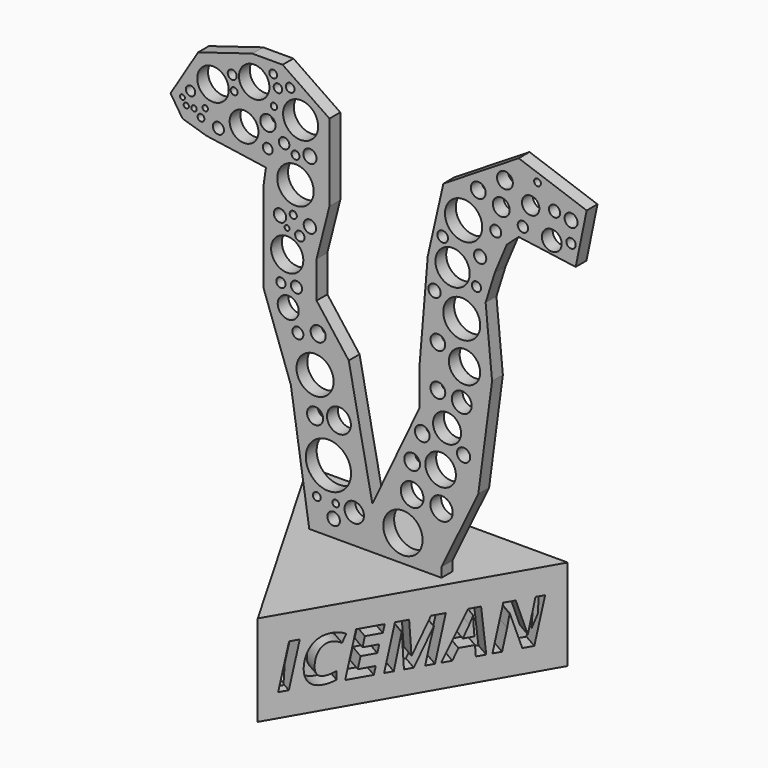
from build123d import *

# Parameters (mm, degrees)
F1_DEPTH     = 27
F2_TEXT_SIZE = 18.3817495487
F3_DEPTH     = 5
F4_TEXT_SIZE = 17.8425786241
F5_DEPTH     = 5
F6_TEXT_SIZE = 19.2699850433
F7_DEPTH     = 5
F9_DEPTH     = 127
F10_R        = 4.2621255768
F10_R_2      = 5.4056711116
F10_R_3      = 4.5113334329
F10_R_4      = 4.6639700848
F10_R_5      = 1.3923551174
F10_R_6      = 0.7328480671
F10_R_7      = 0.767759656
F10_R_8      = 0.8011609316
F10_R_9      = 1
F10_R_10     = 0.8092948289
F10_R_11     = 1.6459744272
F10_R_12     = 2.2704727082
F10_R_13     = 1.0363962707
F10_R_14     = 1.3396073613
F10_R_15     = 5.1942897194
F10_R_16     = 0.9437807842
F10_R_17     = 1.55798255
F10_R_18     = 1.4548048846
F10_R_19     = 1.1783421347
F10_R_20     = 1.9564498282
F10_R_21     = 1.0551848536
F10_R_22     = 1.8332824111
F10_R_23     = 0.7328445764
F10_R_24     = 1.392354505
F10_R_25     = 1.8332749605
F10_R_26     = 4.7727933339
F10_R_27     = 1.3781634382
F10_R_28     = 1.6454183226
F10_R_29     = 3.1159786158
F10_R_30     = 1.6266516452
F10_R_31     = 2.2244104358
F10_R_32     = 5.4998397827
F10_R_33     = 1.9248165419
F10_R_34     = 2.582420861
F10_R_35     = 1.5337907074
F10_R_36     = 2.5096557058
F10_R_37     = 2.1946331857
F10_R_38     = 5.5118577323
F10_R_39     = 5.0853234815
F10_R_40     = 1.5763342381
F10_R_41     = 1.822880463
F10_R_42     = 1.3610571623
F10_R_43     = 1.8260498017
F10_R_44     = 5.4713745158
F10_R_45     = 4.6355846875
F10_R_46     = 2.1776929498
F10_R_47     = 2.1946403477
F10_R_48     = 2.9317995196
F10_R_49     = 4.1461972463
F10_R_50     = 4.5304970367
F10_R_51     = 1.9629433151
F10_R_52     = 3.3115899201
F10_R_53     = 3.3670677037
F10_R_54     = 2.3408899759
F10_R_55     = 5.8192073402
F10_R_56     = 1.8585663298
F10_R_57     = 2.882521964
F10_R_58     = 0.9814695986
F10_R_59     = 1.1548921466
F10_R_60     = 6.7011643118
F10_R_61     = 2.3863964285
F10_R_62     = 3.5387465616
F10_R_63     = 2.3416440081
F10_R_64     = 1.6558003189
F10_R_65     = 2.9317919101
F10_R_66     = 1.3880112598
F10_R_67     = 1.633271575
F10_R_68     = 1.1445034295
F10_R_69     = 1.2597935008
F10_R_70     = 1.2796093116
F11_DEPTH    = 24.2289854638


# Not quite as in the source:
# - Text() gives the source's letters only with a copy of the font that has no kerning and outlines rounded to 1/6400 em; it was checked with that copy


with BuildPart() as f1:
    # F0 (on Top) → F1 (new body)
    with BuildSketch(Plane.XY):
        Polygon((38.5, 22.2279853638), (-38.5, 22.2279853638), (0, -44.4559707276), align=None)
    extrude(amount=F1_DEPTH)

    # F2 (on face) → F3 (cut)
    with BuildSketch(Plane(origin=(0, 22.2279853638, 0), x_dir=(-1, 0, 0), z_dir=(0, 1, 0))):
        with Locations((-35.8188121913, 5.9438663003)):
            Text('ICEMAN', F2_TEXT_SIZE, font='Open Sans', font_style=FontStyle.BOLDITALIC, text_align=(TextAlign.LEFT, TextAlign.BOTTOM))
    extrude(amount=-F3_DEPTH, mode=Mode.SUBTRACT)

    # F4 (on face) → F5 (cut)
    with BuildSketch(Plane(origin=(19.25, -11.1139926819, 0), x_dir=(0.5, 0.8660254038, 0), z_dir=(0.8660254038, -0.5, 0))):
        with Locations((-33.8961333036, 6.8087293766)):
            Text('ICEMAN', F4_TEXT_SIZE, font='Open Sans', font_style=FontStyle.BOLDITALIC, text_align=(TextAlign.LEFT, TextAlign.BOTTOM))
    extrude(amount=-F5_DEPTH, mode=Mode.SUBTRACT)

    # F6 (on face) → F7 (cut)
    with BuildSketch(Plane(origin=(-19.25, -11.1139926819, 0), x_dir=(0.5, -0.8660254038, 0), z_dir=(-0.8660254038, -0.5, 0))):
        with Locations((-36.8695035577, 6.037928164)):
            Text('ICEMAN', F6_TEXT_SIZE, font='Open Sans', font_style=FontStyle.BOLDITALIC, text_align=(TextAlign.LEFT, TextAlign.BOTTOM))
    extrude(amount=-F7_DEPTH, mode=Mode.SUBTRACT)

    # F8 (on face) → F9 (join)
    with BuildSketch(Plane.XY.offset(27)):
        Polygon((24.5119661283, -2), (26.821367205, 2), (-26.821367205, 2), (-24.5119661283, -2), align=None)
        Polygon((-24.5119661283, -2), (-26.821367205, 2), (-63.5, 2), (-63.5, -2), align=None)
        Polygon((63.5, -2), (63.5, 2), (26.821367205, 2), (24.5119661283, -2), align=None)
    extrude(amount=F9_DEPTH)

    # F10 (on face) → F11 (cut, through all)
    with BuildSketch(Plane.XZ.offset(2)):
        Polygon((-6.9961682893, 74.7433826327), (0, 39.6281406283), (14.0115426885, 69.2767286858), (14.0115426885, 80.7320252061), (16.4139904082, 109.5864102244), (21.0415814072, 130.002245307), (43.3628968894, 143.8850164413), (63.5, 136.8075311184), (63.5, 154), (-63.5, 154), (-63.5, 27), (-24.5119661283, 27), (-18.7012497336, 27), (-24.1454709321, 62.7660900354), (-32.3118083179, 85.6318250299), (-32.3118083179, 111.7641031742), (-31.5384617157, 117.1001859978), (-49.1888970137, 119.6582242846), (-56.2663897872, 121.8359172344), (-59.8051324487, 127.2801309824), (-51.6387969255, 140.6184881926), (-35.578340292, 145.5182880163), (-26.5953727067, 145.5182880163), (-12.7126025036, 135.9908878803), (-12.7126025036, 113.1251528859), (-16.5235567838, 98.1535390019), (-16.5235567838, 87.2650966048), align=None)
        Polygon((63.5, 27), (63.5, 136.8075311184), (60.2399893105, 121.0192814469), (43.3398403498, 123.3614778514), (39.8241505027, 120.2026456594), (36.2854078412, 111.7641031742), (33.5632935166, 103.0533388257), (35.4687720537, 83.181925118), (31.3856042922, 52.4220652878), (20.4971581697, 29.8285391182), (20.4971581697, 27), (24.5119661283, 27), align=None)
        with Locations((-38.0282402039, 125.6468743086)):
            Circle(F10_R)
        with Locations((-22.7876920253, 115.4174953699)):
            Circle(F10_R_2)
        with Locations((-35.0095592439, 138.3334994316)):
            Circle(F10_R_3)
        with Locations((-47.2314283252, 133.7502896786)):
            Circle(F10_R_4)
        with Locations((-53.8856498897, 129.825308919)):
            Circle(F10_R_5)
        with Locations((-56.289114058, 127.4218410254)):
            Circle(F10_R_6)
        with Locations((-55.1446080208, 125.5906224251)):
            Circle(F10_R_7)
        with Locations((-52.855592221, 125.5906224251)):
            Circle(F10_R_8)
        with Locations((-50.7757468588, 123.8280911813)):
            Circle(F10_R_9)
        with Locations((-49.5365224779, 126.7351359129)):
            Circle(F10_R_10)
        with Locations((-45.6290878356, 122.7742433548)):
            Circle(F10_R_11)
        with Locations((-30.9507530183, 128.9134025574)):
            Circle(F10_R_12)
        with Locations((-40.952719748, 133.9455246925)):
            Circle(F10_R_13)
        with Locations((-41.5249727666, 138.0657553673)):
            Circle(F10_R_14)
        with Locations((-21.2599616498, 132.8336596489)):
            Circle(F10_R_15)
        with Locations((-29.1642993689, 133.8310837746)):
            Circle(F10_R_16)
        with Locations((-26.1487066746, 125.1949816942)):
            Circle(F10_R_17)
        with Locations((-30.9977401048, 122.22982198)):
            Circle(F10_R_18)
        with Locations((-22.7550584823, 123.1871619821)):
            Circle(F10_R_19)
        with Locations((-18.5100417584, 124.2783516645)):
            Circle(F10_R_20)
        with Locations((-23.4417635947, 107.3929667473)):
            Circle(F10_R_21)
        with Locations((-27.3708961904, 105.9455424547)):
            Circle(F10_R_22)
        with Locations((-25.2729747444, 103.3871918917)):
            Circle(F10_R_23)
        with Locations((-21.4961022139, 102.4715900421)):
            Circle(F10_R_24)
        with Locations((-18.5100417584, 105.9455424547)):
            Circle(F10_R_25)
        with Locations((-25.2320673317, 96.4735969901)):
            Circle(F10_R_26)
        with Locations((-27.1041858941, 88.508605957)):
            Circle(F10_R_27)
        with Locations((-22.4821474403, 88.8349339366)):
            Circle(F10_R_28)
        with Locations((-24.9265227467, 82.7239975333)):
            Circle(F10_R_29)
        with Locations((-22.0703296363, 77.014490962)):
            Circle(F10_R_30)
        with Locations((-16.0656664521, 78.7518918514)):
            Circle(F10_R_31)
        with Locations((-16.982305795, 67.7522048354)):
            Circle(F10_R_32)
        with Locations((58.8789321482, 132.7243596315)):
            Circle(F10_R_33)
        with Locations((46.9016432762, 132.7243596315)):
            Circle(F10_R_34)
        with Locations((44.6018800139, 126.4301240444)):
            Circle(F10_R_35)
        with Locations((38.1908863783, 129.4578313828)):
            Circle(F10_R_36)
        with Locations((31.3856042922, 131.6355168819)):
            Circle(F10_R_37)
        with Locations((27.0302277058, 122.3803386092)):
            Circle(F10_R_38)
        with Locations((23.7636920065, 109.0419888496)):
            Circle(F10_R_39)
        with Locations((20.8356492221, 116.1233410239)):
            Circle(F10_R_40)
        with Locations((18.4105243534, 101.2088209391)):
            Circle(F10_R_41)
        with Locations((30.8411829174, 106.3198745251)):
            Circle(F10_R_42)
        with Locations((31.9300293922, 114.4862100482)):
            Circle(F10_R_43)
        with Locations((26.4858044684, 96.5202748775)):
            Circle(F10_R_44)
        with Locations((27.3024383932, 84.2707753181)):
            Circle(F10_R_45)
        with Locations((19.4083154202, 88.0817249417)):
            Circle(F10_R_46)
        with Locations((19.4083154202, 75.5600109696)):
            Circle(F10_R_47)
        with Locations((26.4858044684, 74.7433826327)):
            Circle(F10_R_48)
        with Locations((22.1304260194, 66.5770471096)):
            Circle(F10_R_49)
        with Locations((14.7807244211, 62.7660900354)):
            Circle(F10_R_46)
        with Locations((20.224949345, 55.1441758871)):
            Circle(F10_R_50)
        with Locations((27.0302277058, 61.1328221858)):
            Circle(F10_R_51)
        with Locations((20.4971581697, 45.0723655522)):
            Circle(F10_R_52)
        with Locations((11.7864022031, 45.8889976144)):
            Circle(F10_R_53)
        with Locations((11.7864022031, 54.4524346571)):
            Circle(F10_R_54)
        with Locations((9.0642916039, 35.000551492)):
            Circle(F10_R_55)
        with Locations((-11.4824660122, 32.0032462478)):
            Circle(F10_R_56)
        with Locations((-5.3715305403, 35.6698036194)):
            Circle(F10_R_57)
        with Locations((-10.8636720106, 36.1962169409)):
            Circle(F10_R_58)
        with Locations((-16.445659101, 36.1962169409)):
            Circle(F10_R_59)
        with Locations((-13.0102001131, 45.4472973943)):
            Circle(F10_R_60)
        with Locations((-16.982305795, 57.0580735803)):
            Circle(F10_R_61)
        with Locations((-9.9012590945, 58.1392049789)):
            Circle(F10_R_62)
        with Locations((39.2797291279, 136.8075311184)):
            Circle(F10_R_63)
        with Locations((48.9316209755, 139.3908824985)):
            Circle(F10_R_9)
        with Locations((53.9791323245, 133.5409879684)):
            Circle(F10_R_64)
        with Locations((53.1625002623, 125.6468743086)):
            Circle(F10_R_65)
        with Locations((58.8789321482, 126.7357170582)):
            Circle(F10_R_66)
        with Locations((36.5576185286, 122.6525455713)):
            Circle(F10_R_67)
        with Locations((-29.3931998312, 142.185986042)):
            Circle(F10_R_68)
        with Locations((-27.981987223, 138.944581151)):
            Circle(F10_R_69)
        with Locations((-24.3573691696, 140.2403116226)):
            Circle(F10_R_70)
    extrude(amount=-F11_DEPTH, mode=Mode.SUBTRACT)


solid = f1.part
